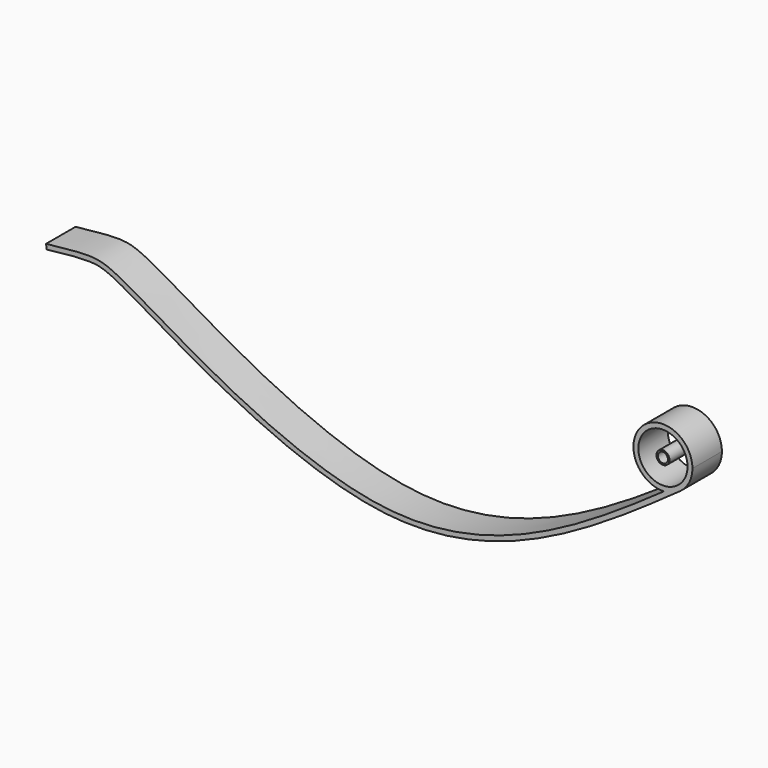
from build123d import *

# Parameters (mm, degrees)
F0_R     = 8
F0_R_2   = 6.1150002293
F1_DEPTH = 45


# Not quite as in the source:
# - the dataset's text gives a spline's control points without its knots; the knots are read off the source's solid


with BuildPart() as f1:
    # F0 (on Front) → F1 (new body)
    with BuildSketch(Plane.XZ):
        Circle(F0_R)
        Circle(F0_R_2, mode=Mode.SUBTRACT)
    extrude(amount=F1_DEPTH)


with BuildPart() as f1b:
    # F0 (on Front) → F1, piece 2 (new body)
    with BuildSketch(Plane.XZ):
        with BuildLine():
            ThreePointArc((36, 0), (-25.8493808233, 25.0561272157), (1.1216938305, -35.9825207976))
            ThreePointArc((1.1216938305, -35.9825207976), (11.4894376417, -34.1173390328), (20.8734070894, -29.33088605))
            ThreePointArc((20.8734070894, -29.33088605), (31.9956454476, -16.5008688375), (36, 0))
        make_face()
        with BuildLine():
            ThreePointArc((17.3945059078, -24.4424050417), (-26.663037873, 13.7507240312), (30, 0))
            ThreePointArc((30, 0), (26.663037873, -13.7507240312), (17.3945059078, -24.4424050417))
        make_face(mode=Mode.SUBTRACT)
        with BuildLine():
            ThreePointArc((20.8734070894, -29.33088605), (11.4894376417, -34.1173390328), (1.1216938305, -35.9825207976))
            add(Edge.make_bspline(
                [(-335.4028873897, -164.5892359471), (-211.660023101, -178.1492344891), (-104.9968000053, -110.9002326589), (1.1216938305, -35.9825207976)],
                knots=[0.6260346146, 0.6260346146, 0.6260346146, 0.6260346146, 0.9818120521, 0.9818120521, 0.9818120521, 0.9818120521], degree=3))
            add(Edge.make_bspline(
                [(-752.9035652414, -15.1577310849), (-733.5255763767, -12.913793992), (-696.8907544765, -8.6504785513), (-653.5982811894, -20.375212445), (-460.8298083922, -150.8446949935), (-335.4028873897, -164.5892359471)],
                knots=[0, 0, 0, 0, 0.1398221538, 0.2654152866, 0.6260346146, 0.6260346146, 0.6260346146, 0.6260346146], degree=3))
            Line((-752.9035652414, -15.1577310849), (-752.2133877406, -21.1179034832))
            add(Edge.make_bspline(
                [(-752.2133877406, -21.1179034832), (-747.8819401783, -20.6163294592), (-741.4054657906, -19.8655808623), (-732.9816784766, -18.9535340135), (-726.813295097, -18.3352940539), (-720.8388549156, -17.8040416904), (-716.0599042092, -17.4512810499), (-712.3803835531, -17.2332747887), (-709.6987601974, -17.1043494034), (-707.1014925809, -17.0124208139), (-704.5952040028, -16.9598034746), (-702.5880681745, -16.9505287011), (-701.0350684421, -16.964842098), (-699.8970408217, -16.9866530163), (-698.7894719832, -17.0197776915), (-697.3503439127, -17.0801856153), (-695.6145720888, -17.1881586484), (-693.6081111097, -17.3760989816), (-690.9987201877, -17.7137085003), (-688.4303551952, -18.1965971676), (-685.783769195, -18.8632180172), (-683.7311833316, -19.4666860211), (-681.5842178154, -20.1854270516), (-678.5630496726, -21.313191571), (-674.4319558802, -23.0694636499), (-669.6906989632, -25.3570452936), (-665.4545548363, -27.5422026086), (-662.0371669654, -29.366825564), (-658.3586470674, -31.3863523905), (-653.1171965191, -34.3258182347), (-645.9572814799, -38.4368276945), (-636.4561652376, -43.9898284169), (-626.1041259099, -50.0858658916), (-614.9566716437, -56.6494574293), (-603.0676587769, -63.605904565), (-590.4899301352, -70.8810113959), (-577.2756616032, -78.4009117992), (-558.876827584, -88.6556534453), (-534.5446264486, -101.7182022108), (-503.6195372905, -117.1969794879), (-471.3712759239, -131.8930877898), (-443.7277935087, -142.9984439362), (-421.3481501748, -150.903183668), (-404.4796901539, -156.2678433326), (-387.575931455, -160.9941300803), (-373.5000999922, -164.3381791949), (-362.2697054677, -166.6187803013), (-353.868007044, -168.1223279176), (-346.8891204735, -169.1948451716), (-341.3225548845, -169.9397145241), (-337.1565441963, -170.4406244587), (-333.0006313018, -170.8823459866), (-327.476337024, -171.3922432213), (-320.6011986985, -171.8831865525), (-312.3992482092, -172.242591318), (-301.5266846141, -172.4218287997), (-288.0534050114, -172.0952904497), (-272.0683532648, -170.8610068572), (-256.2607402739, -168.8232870132), (-235.4124158177, -165.0875255318), (-209.7641163299, -158.6064022713), (-179.585483077, -148.2471492799), (-149.9383621316, -135.6198797987), (-120.7505892392, -121.0345206642), (-91.9481020771, -104.7971337372), (-63.4566763981, -87.2106556503), (-25.7851652267, -62.364087001), (2.2202830336, -42.6054339529), (20.8734070894, -29.33088605)],
                knots=[0, 0, 0, 0, 0.03125, 0.046875, 0.0625, 0.078125, 0.09375, 0.1015625, 0.109375, 0.1171875, 0.125, 0.1328125, 0.13671875, 0.140625, 0.14453125, 0.1484375, 0.15625, 0.1640625, 0.171875, 0.1875, 0.1953125, 0.203125, 0.2109375, 0.21875, 0.234375, 0.25, 0.2578125, 0.265625, 0.2734375, 0.28125, 0.296875, 0.3125, 0.328125, 0.34375, 0.359375, 0.375, 0.390625, 0.40625, 0.4375, 0.46875, 0.5, 0.53125, 0.546875, 0.5625, 0.578125, 0.59375, 0.6015625, 0.609375, 0.6171875, 0.62109375, 0.625, 0.62890625, 0.6328125, 0.640625, 0.6484375, 0.65625, 0.671875, 0.6875, 0.703125, 0.71875, 0.75, 0.78125, 0.8125, 0.84375, 0.875, 0.90625, 0.9375, 1, 1, 1, 1], degree=3))
        make_face()
    extrude(amount=F1_DEPTH)


solid = Compound([f1.part, f1b.part])
